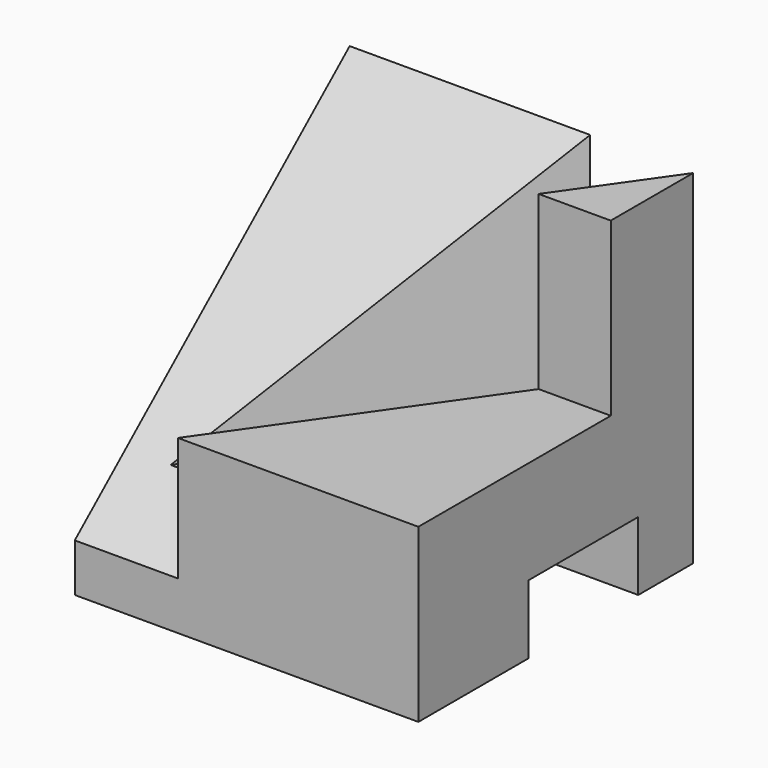
from build123d import *

# Parameters (mm, degrees)
F0_W     = 50
F0_H     = 50
F1_DEPTH = 50
F2_W     = 20
F2_H     = 10
F3_DEPTH = 30
F5_DEPTH = 25
F7_DEPTH = 35
F9_REACH = 115.9479483752


with BuildPart() as f1:
    # F0 (on Top) → F1 (new body)
    with BuildSketch(Plane.XY):
        with Locations((25, 25)):
            Rectangle(F0_W, F0_H)
    extrude(amount=F1_DEPTH)

    # F2 (on face) → F3 (cut)
    with BuildSketch(Plane.YZ.offset(50)):
        with Locations((30, 5)):
            Rectangle(F2_W, F2_H)
    extrude(amount=-F3_DEPTH, mode=Mode.SUBTRACT)

    # F4 (on face) → F5 (cut)
    with BuildSketch(Plane.XY.offset(50)):
        Polygon((50, 35), (39.5, 35), (15, 0), (50, 0), align=None)
    extrude(amount=-F5_DEPTH, mode=Mode.SUBTRACT)

    # F6 (on face) → F7 (cut)
    with BuildSketch(Plane.XY.offset(50)):
        Polygon((39.5, 35), (50, 50), (35, 50), (0, 0), (15, 0), align=None)
    extrude(amount=-F7_DEPTH, mode=Mode.SUBTRACT)

    f9_end = Plane(origin=(37.75, 32.5, 27.5), x_dir=(-0.5734623444, -0.8192319205, 0), z_dir=(-0.8192319205, 0.5734623444, 0))
    # F8 (on face) → F9 (cut, up to a plane its end follows)
    with BuildSketch(Plane(origin=(0, 0, 0), x_dir=(0, -1, 0), z_dir=(-1, 0, 0))):
        Polygon((-50, 50), (0, 7), (0, 15), (0, 50), align=None)
    f9_long = extrude(amount=-F9_REACH, mode=Mode.PRIVATE)
    add(split(f9_long, bisect_by=f9_end, keep=Keep.TOP, mode=Mode.PRIVATE), mode=Mode.SUBTRACT)


solid = f1.part
